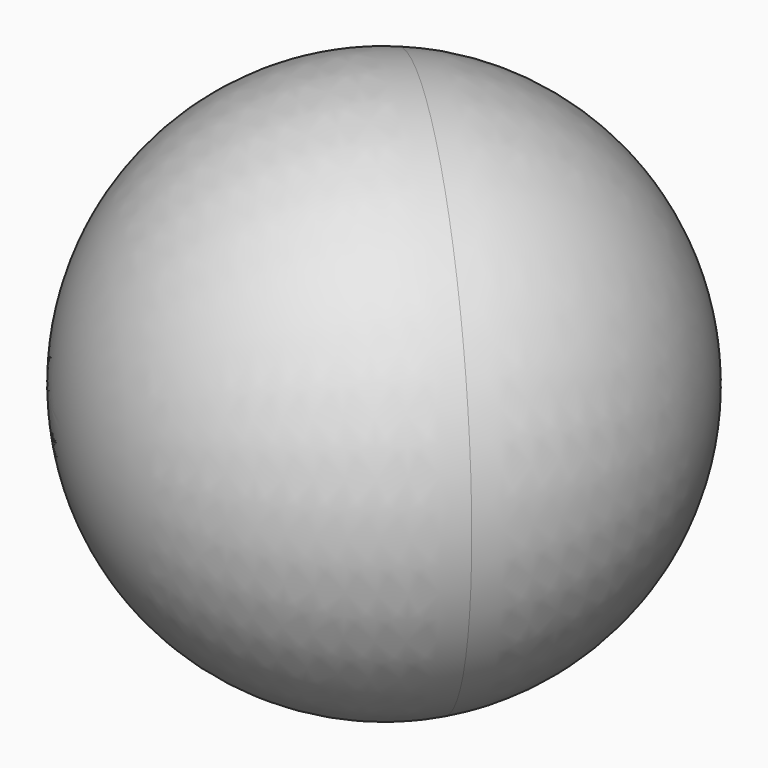
from build123d import *


with BuildPart() as f1:
    # F0 (on Top) → F1 (revolve)
    with BuildSketch(Plane.XY):
        with BuildLine():
            Line((-0.0645753372, 0.0544318257), (-14.2066145431, -15.2573901879))
            ThreePointArc((-14.2066145431, -15.2573901879), (1.9574152389, -20.7553457621), (16.8085772453, -12.3323794586))
            ThreePointArc((16.8085772453, -12.3323794586), (20.747254181, 2.0413956186), (14.0826575843, 15.371877162))
            Line((14.0826575843, 15.371877162), (-0.0645753372, 0.0544318257))
        make_face()
    revolve(axis=Axis((-0.0619784794, 0.0572434871, 0), (0.6784885966, 0.734610934, 0)))


solid = f1.part
